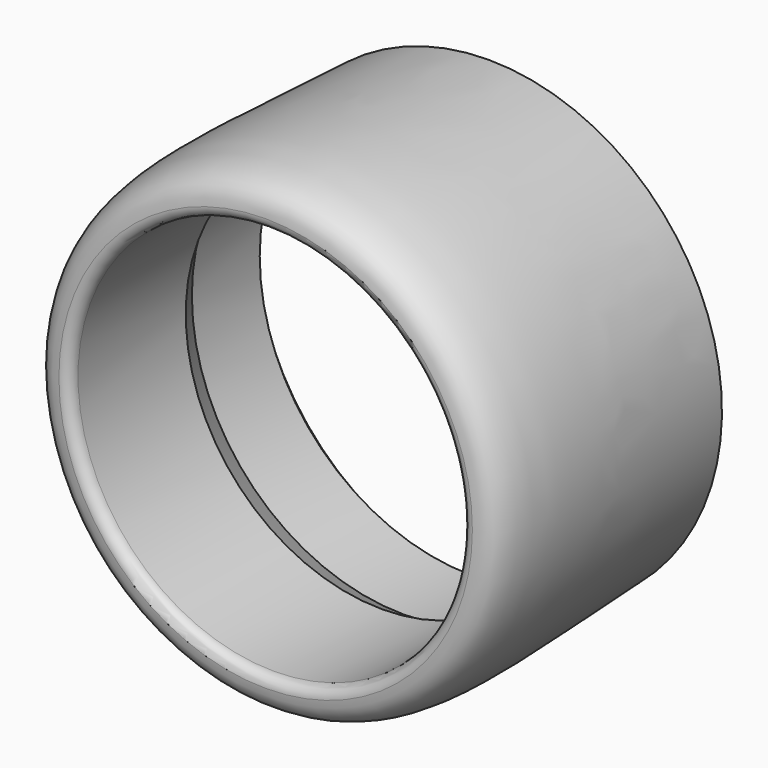
from build123d import *

# Parameters (mm, degrees)
F2_R    = 0.99999
F3_SIZE = 1.99999


# Not quite as in the source:
# - a fillet or chamfer is up to 0.001 mm smaller than in the source, because OpenCascade refuses the exact size


with BuildPart() as f1:
    # F0 (on Right) → F1 (revolve)
    with BuildSketch(Plane.YZ):
        with BuildLine():
            Line((-16.3, 18.5), (-2.5980762114, 18.5))
            Line((-2.5980762114, 18.5), (0, 20))
            Line((0, 20), (10, 20))
            Line((10, 20), (10, 22))
            add(Edge.make_bspline(
                [(-16.3, 19.5), (-16.2997247245, 20.0612064454), (-15.716548184, 23.7883678508), (-1.1838388212, 22.3861274398), (10, 22)],
                knots=[0, 0, 0, 0, 0.2291458751, 1, 1, 1, 1], degree=3))
            Line((-16.3, 19.5), (-16.3, 18.5))
        make_face()
    revolve(axis=Axis((0, -8.15, 0), (0, -1, 0)))

    # F2 (radius 1 in the source; OpenCascade refuses exactly that, so slightly less here)
    f2_edges = [f1.edges().sort_by_distance(p)[0] for p in [
        (0, -16.3, -18.5),
    ]]
    fillet(f2_edges, radius=F2_R)

    # F3 (size 2 in the source; OpenCascade refuses exactly that, so slightly less here)
    f3_edges = [f1.edges().sort_by_distance(p)[0] for p in [
        (0, 10, -20),
    ]]
    chamfer(f3_edges, length=F3_SIZE)


solid = f1.part
